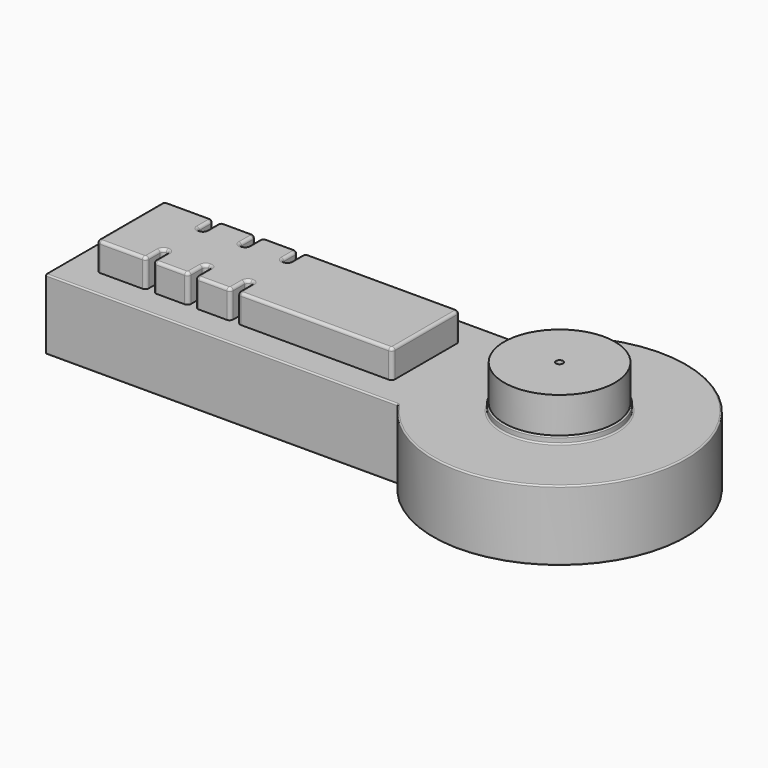
from build123d import *

# Parameters (mm, degrees)
F0_W      = 250
F0_H      = 100
F1_DEPTH  = 50
F3_DEPTH  = 20
F4_R      = 40.3789988007
F5_DEPTH  = 5
F6_R      = 2.5
F7_DEPTH  = 5
F8_R      = 1
F9_R      = 2.49999
F10_R     = 2
F11_DEPTH = 25.4


# Not quite as in the source:
# - a fillet or chamfer is up to 0.001 mm smaller than in the source, because OpenCascade refuses the exact size


with BuildPart() as f1:
    # F0 (on Top) → F1 (new body)
    with BuildSketch(Plane.XY):
        with Locations((125, 50)):
            Rectangle(F0_W, F0_H)
        with BuildLine():
            Line((250, 100), (250, 0))
            ThreePointArc((250, 0), (415.1387818866, 50), (250, 100))
        make_face()
    extrude(amount=F1_DEPTH)

    # F2 (on face) → F3 (join)
    with BuildSketch(Plane.XY.offset(50)):
        Polygon((55, 80), (20, 80), (20, 20), (55, 20), (55, 35), (60, 35), (60, 20), (85, 20), (85, 35), (90, 35), (90, 20), (115, 20), (115, 35), (120, 35), (120, 20), (230, 20), (230, 80), (120, 80), (120, 65), (115, 65), (115, 80), (90, 80), (90, 65), (85, 65), (85, 80), (60, 80), (60, 65), (55, 65), align=None)
    extrude(amount=F3_DEPTH)

    # F4 (on face) → F5 (join)
    with BuildSketch(Plane.XY.offset(50)):
        with Locations((325, 50)):
            Circle(F4_R)
    extrude(amount=F5_DEPTH)

    # F6 (on face) → F7 (join)
    with BuildSketch(Plane.XY.offset(55)):
        with Locations((325, 50)):
            Circle(F6_R)
    extrude(amount=F7_DEPTH)

    # F8
    f8_edges = [f1.edges().sort_by_distance(p)[0] for p in [
        (250, 0, 25),
        (250, 100, 25),
        (415.138782, 50, 0),
        (415.138782, 50, 50),
        (284.621001, 50, 55),
        (284.621001, 50, 50),
        (125, 100, 0),
        (125, 100, 50),
        (125, 0, 0),
        (125, 0, 50),
    ]]
    fillet(f8_edges, radius=F8_R)

    # F9 (radius 2.5 in the source; OpenCascade refuses exactly that, so slightly less here)
    f9_edges = [f1.edges().sort_by_distance(p)[0] for p in [
        (55, 35, 60),
        (55, 20, 60),
        (60, 35, 60),
        (60, 20, 60),
        (85, 20, 60),
        (90, 35, 60),
        (90, 20, 60),
        (115, 20, 60),
        (120, 35, 60),
        (120, 20, 60),
        (85, 35, 60),
        (115, 35, 60),
        (55, 65, 60),
        (55, 80, 60),
        (85, 65, 60),
        (85, 80, 60),
        (115, 65, 60),
        (115, 80, 60),
        (60, 65, 60),
        (60, 80, 60),
        (90, 65, 60),
        (90, 80, 60),
        (120, 65, 60),
        (120, 80, 60),
        (20, 80, 60),
        (20, 20, 60),
        (230, 80, 60),
        (230, 20, 60),
    ]]
    fillet(f9_edges, radius=F9_R)

    # F10
    f10_edges = [f1.edges().sort_by_distance(p)[0] for p in [
        (175, 80, 70),
        (230, 50, 70),
        (37.5, 80, 70),
        (54.26777, 79.26777, 70),
        (20.73223, 79.26777, 70),
        (55, 72.5, 70),
        (20, 50, 70),
        (55.73223, 65.73223, 70),
        (20.73223, 20.73223, 70),
        (57.5, 65, 70),
        (37.5, 20, 70),
        (59.26777, 65.73223, 70),
        (54.26777, 20.73223, 70),
        (60, 72.5, 70),
        (55, 27.5, 70),
        (60.73223, 79.26777, 70),
        (55.73223, 34.26777, 70),
        (72.5, 80, 70),
        (57.5, 35, 70),
        (84.26777, 79.26777, 70),
        (59.26777, 34.26777, 70),
        (85, 72.5, 70),
        (60, 27.5, 70),
        (85.73223, 65.73223, 70),
        (60.73223, 20.73223, 70),
        (87.5, 65, 70),
        (72.5, 20, 70),
        (89.26777, 65.73223, 70),
        (84.26777, 20.73223, 70),
        (90, 72.5, 70),
        (85, 27.5, 70),
        (90.73223, 79.26777, 70),
        (85.73223, 34.26777, 70),
        (102.5, 80, 70),
        (87.5, 35, 70),
        (114.26777, 79.26777, 70),
        (89.26777, 34.26777, 70),
        (115, 72.5, 70),
        (90, 27.5, 70),
        (115.73223, 65.73223, 70),
        (90.73223, 20.73223, 70),
        (117.5, 65, 70),
        (102.5, 20, 70),
        (119.26777, 65.73223, 70),
        (114.26777, 20.73223, 70),
        (120, 72.5, 70),
        (115, 27.5, 70),
        (120.73223, 79.26777, 70),
        (115.73223, 34.26777, 70),
        (117.5, 35, 70),
        (229.26777, 79.26777, 70),
        (119.26777, 34.26777, 70),
        (120, 27.5, 70),
        (229.26777, 20.73223, 70),
        (120.73223, 20.73223, 70),
        (175, 20, 70),
    ]]
    fillet(f10_edges, radius=F10_R)

    # F11 (add): a face of the model
    f11_faces = [f1.faces().sort_by_distance(p)[0] for p in [
        (286.7348074828, 50, 55),
    ]]
    extrude(f11_faces, amount=F11_DEPTH)


solid = f1.part
